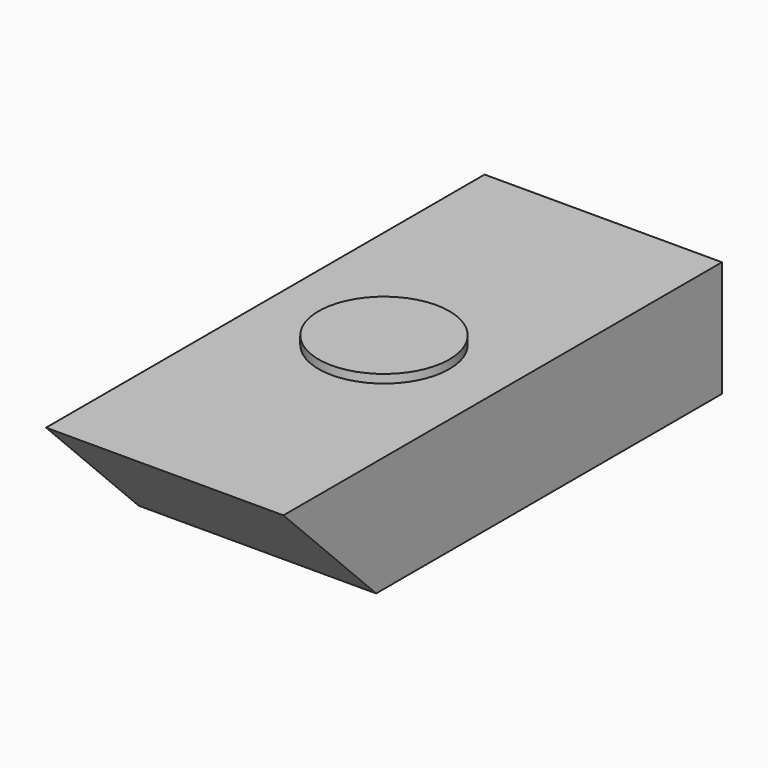
from build123d import *

# Parameters (mm, degrees)
F0_W     = 15.6047875062
F0_H     = 36.0328741372
F1_DEPTH = 7.62
F2_SIZE  = 7.61999
F3_R     = 4.2995581312
F4_DEPTH = 0.5588


# Not quite as in the source:
# - a fillet or chamfer is up to 0.001 mm smaller than in the source, because OpenCascade refuses the exact size


with BuildPart() as f1:
    # F0 (on Top) → F1 (new body)
    with BuildSketch(Plane.XY):
        Rectangle(F0_W, F0_H)
    extrude(amount=F1_DEPTH)

    # F2 (size 7.62 in the source; OpenCascade refuses exactly that, so slightly less here)
    f2_edges = [f1.edges().sort_by_distance(p)[0] for p in [
        (0, -18.016437, 0),
    ]]
    chamfer(f2_edges, length=F2_SIZE)

    # F3 (on face) → F4 (join)
    with BuildSketch(Plane.XY.offset(7.62)):
        Circle(F3_R)
    extrude(amount=F4_DEPTH)


solid = f1.part
